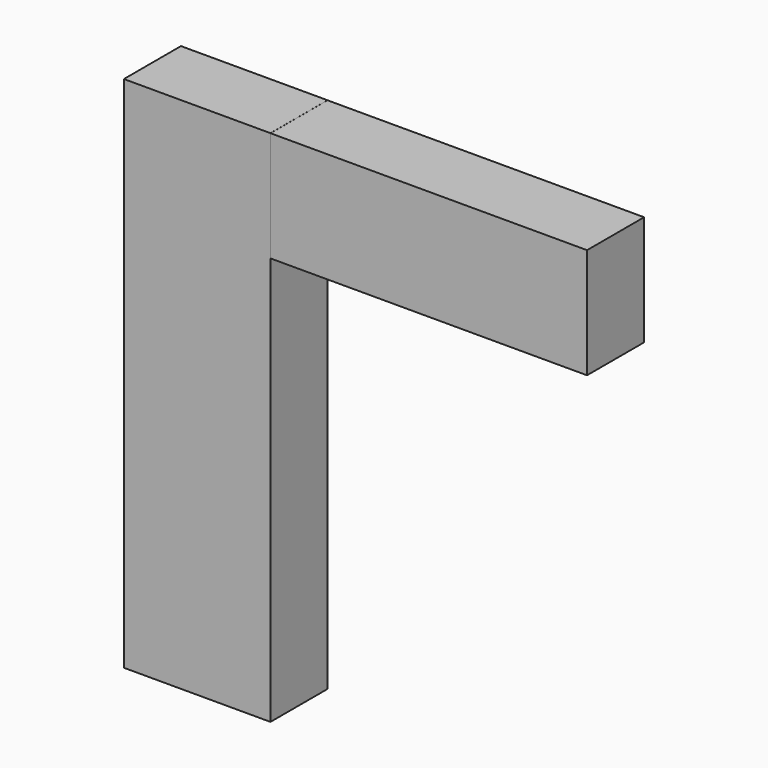
from build123d import *

# Parameters (mm, degrees)
F1_W     = 61.5491271019
F1_H     = 21.3788896799
F2_DEPTH = 13.8399954885
F0_W     = 28.4387171268
F0_H     = 100.5795300007


with BuildPart() as f2:
    # F1 (on Front) → F2 (new body)
    with BuildSketch(Plane.XZ):
        with Locations((44.8790490627, 39.5893901587)):
            Rectangle(F1_W, F1_H)
    extrude(amount=F2_DEPTH)


with BuildPart() as f2b:
    # F0 (on Front) → F2, piece 2 (new body)
    with BuildSketch(Plane.XZ):
        Rectangle(F0_W, F0_H)
    extrude(amount=F2_DEPTH)


solid = Compound([f2.part, f2b.part])
